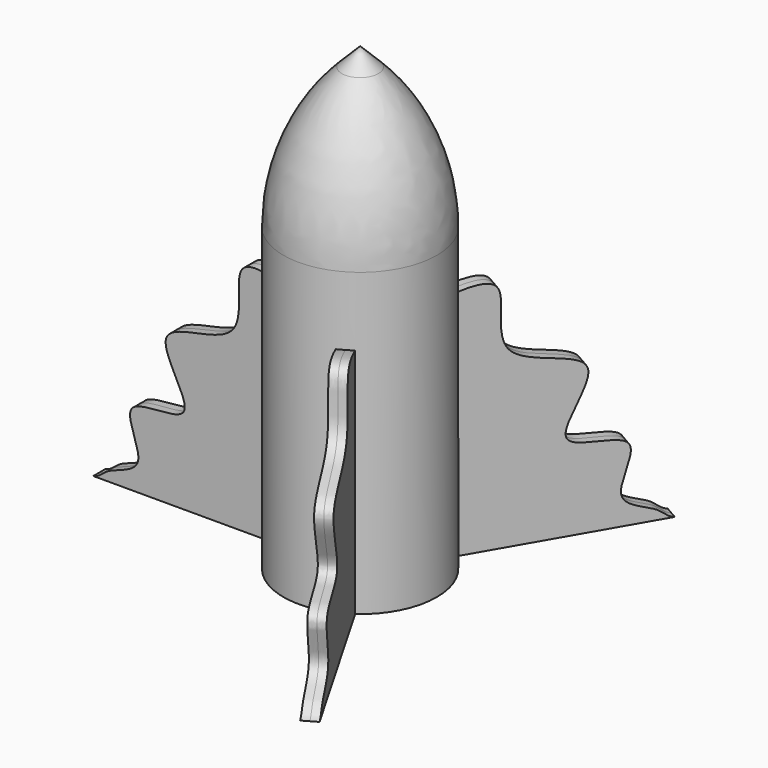
from build123d import *

# Parameters (mm, degrees)
F0_R            = 12.7
F1_DEPTH        = 76.2
F2_SIZE         = 12.7
F3_R            = 33.02
F4_T            = -1.27
F6_DEPTH        = 1.27
F6_COPIES_COUNT = 3


# Not quite as in the source:
# - a feature of the source that left no trace in its solid (it failed there, or was rolled back) is left out
# - a pattern or mirror of a feature is missing from the dataset's text; its kind, count and spacing are read off the source's solid


with BuildPart() as f1:
    # F0 (on Top) → F1 (new body)
    with BuildSketch(Plane.XY):
        Circle(F0_R)
    extrude(amount=F1_DEPTH)

    # F2
    f2_edges = [f1.edges().sort_by_distance(p)[0] for p in [
        (-12.7, 0, 76.2),
    ]]
    chamfer(f2_edges, length=F2_SIZE)

    # F3
    f3_edges = [f1.edges().sort_by_distance(p)[0] for p in [
        (-12.7, 0, 63.5),
    ]]
    fillet(f3_edges, radius=F3_R)

    # F4
    f4_openings = [f1.faces().sort_by_distance(p)[0] for p in [
        (0, 0, 0),
    ]]
    offset(amount=F4_T, openings=f4_openings)

    # F5 (on Front) → F6 (join, symmetric)
    with BuildSketch(Plane.XZ):
        with BuildLine():
            Line((-43.18, 0), (-11.43, 0))
            Line((-11.43, 0), (-11.43, 38.1))
            add(Edge.make_bspline(
                [(-11.43, 38.1), (-14.0398158155, 38.8052379758), (-21.4254245672, 40.7158801474), (-15.9788784795, 25.3635431222), (-37.1308960464, 27.3458822388), (-22.5998042996, 11.213618898), (-41.0016315, 14.671173077), (-32.8964049327, 3.2713549274), (-41.191333005, 2.0523352832), (-41.9971624056, 0.2572525646), (-43.18, 0)],
                knots=[0, 0, 0, 0, 0.1201823933, 0.2593472766, 0.4139037511, 0.5575664377, 0.6914417304, 0.8144088518, 0.9212401283, 1, 1, 1, 1], degree=3))
        make_face()
    f6 = extrude(amount=F6_DEPTH, both=True)

    # F6_copies: F6 ×3 about axis
    f6_copies_axis = Axis((0, 0, 0), (0, 0, 1))
    for i in range(1, F6_COPIES_COUNT):
        add(f6.rotate(f6_copies_axis, i * 360 / F6_COPIES_COUNT))


solid = f1.part
